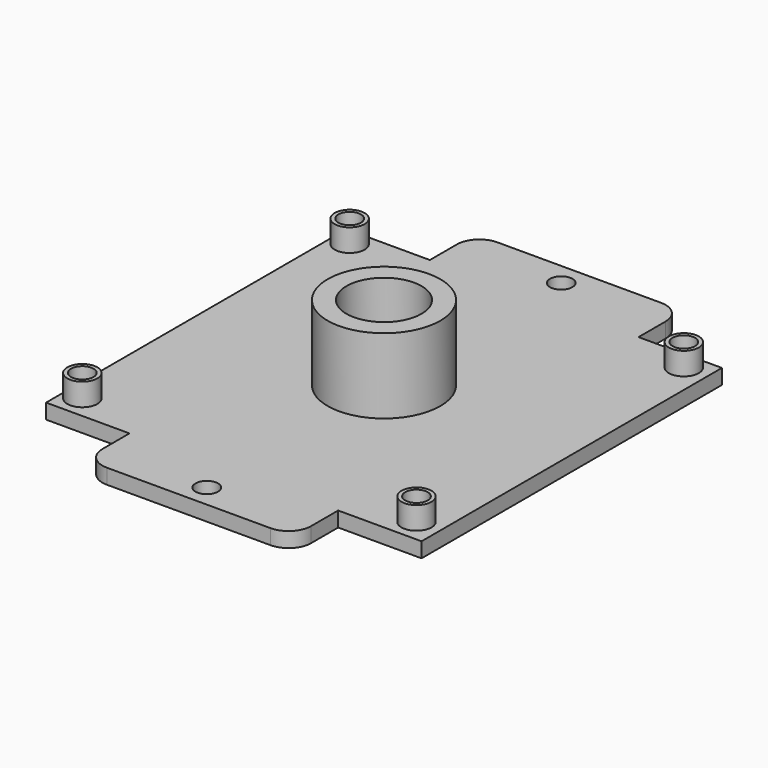
from build123d import *

# Parameters (mm, degrees)
F0_W      = 50
F0_H      = 50
F1_DEPTH  = 2
F2_R      = 2
F3_DEPTH  = 3
F4_R      = 1.5
F5_DEPTH  = 3
F7_DEPTH  = 2
F8_R      = 1.5
F9_DEPTH  = 25
F10_R     = 7.5
F11_DEPTH = 10
F12_R     = 5
F13_DEPTH = 10
F14_DEPTH = 7.7


# Not quite as in the source:
# - a pattern or mirror of a feature is missing from the dataset's text; its kind, count and spacing are read off the source's solid
# - a feature names something its author has since deleted; it is built from what else it names


with BuildPart() as f1:
    # F0 (on Top) → F1 (new body)
    with BuildSketch(Plane.XY):
        Rectangle(F0_W, F0_H)
    extrude(amount=F1_DEPTH)

    # F2 (on face) → F3 (join)
    with BuildSketch(Plane.XY.offset(2)):
        with Locations((-22.6419584364, -21.9144617685)):
            Circle(F2_R)
        with Locations((21.8580415636, -21.9144617685)):
            Circle(F2_R)
        with Locations((21.8580415636, 22.5855382315)):
            Circle(F2_R)
    f3 = extrude(amount=F3_DEPTH)

    # F3_copies: F3 across plane
    add(f3.mirror(Plane.ZX.offset(0.335538)))

    # F4 (on face) → F5 (cut)
    with BuildSketch(Plane.XY.offset(5)):
        with Locations((-22.6419584364, 22.5855382315)):
            Circle(F4_R)
        with Locations((21.8580415636, -21.9144617685)):
            Circle(F4_R)
        with Locations((21.8580415636, 22.5855382315)):
            Circle(F4_R)
        with Locations((-22.6419584364, -21.9144617685)):
            Circle(F4_R)
    extrude(amount=-F5_DEPTH, mode=Mode.SUBTRACT)

    # F6 (on Top) → F7 (join)
    with BuildSketch(Plane.XY):
        with BuildLine():
            ThreePointArc((13.8950906601, 29.5), (13.0164110037, 31.6213203436), (10.8950906601, 32.5))
            Line((10.8950906601, 32.5), (-10.8950906601, 32.5))
            ThreePointArc((-10.8950906601, 32.5), (-13.0164110037, 31.6213203436), (-13.8950906601, 29.5))
            Line((-13.8950906601, 29.5), (-13.8950906601, 25))
            Line((-13.8950906601, 25), (13.8950906601, 25))
            Line((13.8950906601, 25), (13.8950906601, 29.5))
        make_face()
        with BuildLine():
            Line((13.8950906601, -25), (-13.8950906601, -25))
            Line((-13.8950906601, -25), (-13.8950906601, -29.5))
            ThreePointArc((-13.8950906601, -29.5), (-13.0164110037, -31.6213203436), (-10.8950906601, -32.5))
            Line((-10.8950906601, -32.5), (10.8950906601, -32.5))
            ThreePointArc((10.8950906601, -32.5), (13.0164110037, -31.6213203436), (13.8950906601, -29.5))
            Line((13.8950906601, -29.5), (13.8950906601, -25))
        make_face()
    extrude(amount=F7_DEPTH)

    # F8 (on face) → F9 (cut)
    with BuildSketch(Plane.XY.offset(2)):
        with Locations((0, 29.5)):
            Circle(F8_R)
        with Locations((0, -29.5)):
            Circle(F8_R)
    extrude(amount=-F9_DEPTH, mode=Mode.SUBTRACT)

    # F10 (on face) → F11 (join)
    with BuildSketch(Plane.XY.offset(2)):
        Circle(F10_R)
    extrude(amount=F11_DEPTH)

    # F12 (on face) → F13 (cut)
    with BuildSketch(Plane.XY.offset(12)):
        Circle(F12_R)
    extrude(amount=-F13_DEPTH, mode=Mode.SUBTRACT)

    # F14 (cut): faces of the model
    f14_faces = [f1.faces().sort_by_distance(p)[0] for p in [
        (-22.6419584364, -21.9144617685, 2),
        (-22.6419584364, 22.5855382315, 2),
        (21.8580415636, 22.5855382315, 2),
        (21.8580415636, -21.9144617685, 2),
    ]]
    extrude(f14_faces, amount=-F14_DEPTH, mode=Mode.SUBTRACT)


solid = f1.part
